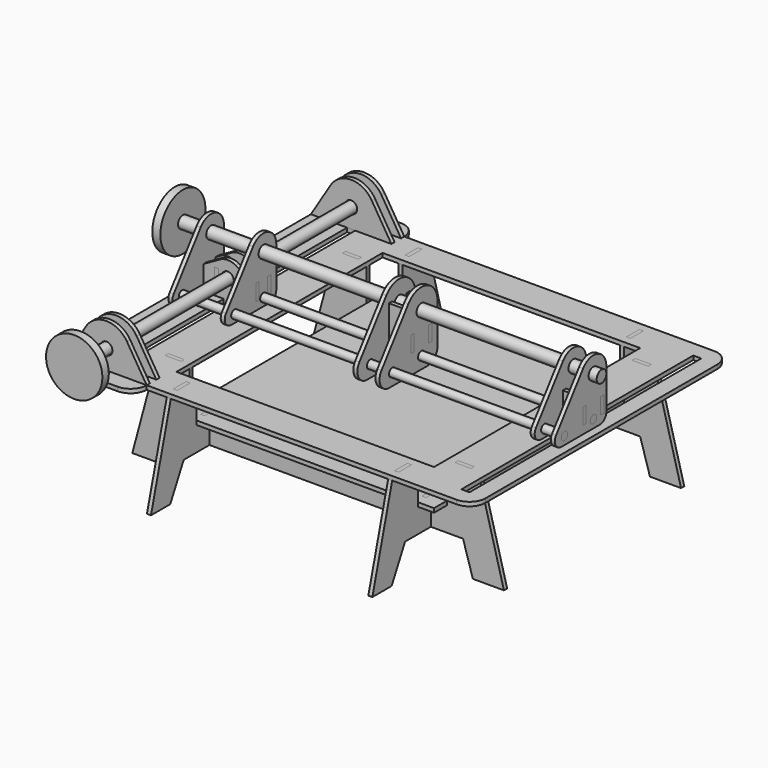
from build123d import *

# Parameters (mm, degrees)
F0_W           = 203.2
F0_H           = 203.2
F1_DEPTH       = 3.175
F3_W           = 203.2
F3_H           = 203.2
F4_DEPTH       = 3.175
F6_DEPTH       = 3.175
F10_DEPTH      = 3.175
F14_DEPTH      = 3.175
F7_W           = 6.35
F7_H           = 228.6
F16_DEPTH      = 8.128
F18_R          = 4.7625
F19_DEPTH      = 3.175
F25_R          = 3.175
F25_R_2        = 4.7625
F26_DEPTH      = 3.175
F30_R          = 4.7625
F31_DEPTH      = 3.175
F34_R          = 3.175
F34_R_2        = 4.7625
F35_DEPTH      = 3.175
F38_R          = 3.175
F39_DEPTH      = 146.05
F39_DEPTH_BACK = 158.75
F41_R          = 3.302
F41_R_2        = 4.7625
F42_DEPTH      = 3.175
F44_R          = 4.7625
F45_DEPTH      = 152.4
F45_DEPTH_BACK = 177.8
F46_R          = 4.4516956425
F47_DEPTH      = 152.4
F47_DEPTH_BACK = 133.35
F49_DEPTH      = 3.175
F51_R          = 22.225
F51_R_2        = 4.4516956425
F52_DEPTH      = 6.35
F53_R          = 22.225
F53_R_2        = 4.7625
F54_DEPTH      = 6.35
F55_W          = 3.175
F55_H          = 12.7
F56_DEPTH      = 3.175
F61_DEPTH      = 3.175
F63_W          = 3.175
F63_H          = 12.7
F63_W_2        = 12.7
F63_H_2        = 3.175
F64_DEPTH      = 25.4
F65_W          = 12.7
F65_H          = 3.175
F66_DEPTH      = 25.4
F67_W          = 3.175
F67_H          = 6.35
F68_DEPTH      = 25.4
F69_W          = 3.175
F69_H          = 12.7
F70_DEPTH      = 51.054
F71_W          = 3.175
F71_H          = 12.7
F72_DEPTH      = 25.4
F73_W          = 3.175
F73_H          = 12.7
F74_DEPTH      = 25.4
F76_DEPTH      = 25.4


with BuildPart() as f1:
    # F0 (on Top) → F1 (new body)
    with BuildSketch(Plane.XY):
        Rectangle(F0_W, F0_H)
    extrude(amount=-F1_DEPTH)

    # F75 (on face) → F76 (cut)
    with BuildSketch(Plane.XY):
        Polygon((-85.725, 88.9), (-85.725, 93.6625), (-88.9, 93.6625), (-88.9, 88.9), (-93.6625, 88.9), (-93.6625, 85.725), (-88.9, 85.725), (-88.9, 80.9625), (-85.725, 80.9625), (-85.725, 85.725), (-80.9625, 85.725), (-80.9625, 88.9), align=None)
        Polygon((88.9, 85.725), (93.6625, 85.725), (93.6625, 88.9), (88.9, 88.9), (88.9, 93.6625), (85.725, 93.6625), (85.725, 88.9), (80.9625, 88.9), (80.9625, 85.725), (85.725, 85.725), (85.725, 80.9625), (88.9, 80.9625), align=None)
        Polygon((-88.9, -88.9), (-88.9, -93.6625), (-85.725, -93.6625), (-85.725, -88.9), (-80.9625, -88.9), (-80.9625, -85.725), (-85.725, -85.725), (-85.725, -80.9625), (-88.9, -80.9625), (-88.9, -85.725), (-93.6625, -85.725), (-93.6625, -88.9), align=None)
        Polygon((85.725, -93.6625), (88.9, -93.6625), (88.9, -88.9), (93.6625, -88.9), (93.6625, -85.725), (88.9, -85.725), (88.9, -80.9625), (85.725, -80.9625), (85.725, -85.725), (80.9625, -85.725), (80.9625, -88.9), (85.725, -88.9), align=None)
    extrude(amount=-F76_DEPTH, mode=Mode.SUBTRACT)


with BuildPart() as f4:
    # F3 (on offset) → F4 (new body)
    with BuildSketch(Plane.XY.offset(25.4)):
        with BuildLine():
            Line((114.3, 127), (-114.3, 127))
            Line((-114.3, 127), (-139.7, 127))
            ThreePointArc((-139.7, 127), (-148.6802561211, 123.2802561211), (-152.4, 114.3))
            Line((-152.4, 114.3), (-152.4, 101.6))
            Line((-152.4, 101.6), (-152.4, -101.6))
            Line((-152.4, -101.6), (-152.4, -114.3))
            ThreePointArc((-152.4, -114.3), (-148.6802561211, -123.2802561211), (-139.7, -127))
            Line((-139.7, -127), (-114.3, -127))
            Line((-114.3, -127), (114.3, -127))
            Line((114.3, -127), (139.7, -127))
            ThreePointArc((139.7, -127), (148.6802561211, -123.2802561211), (152.4, -114.3))
            Line((152.4, -114.3), (152.4, -101.6))
            Line((152.4, -101.6), (152.4, 101.6))
            Line((152.4, 101.6), (152.4, 114.3))
            ThreePointArc((152.4, 114.3), (148.6802561211, 123.2802561211), (139.7, 127))
            Line((139.7, 127), (114.3, 127))
        make_face()
        Rectangle(F3_W, F3_H, mode=Mode.SUBTRACT)
    extrude(amount=F4_DEPTH)

    # F5 (on face) → F6 (join)
    with BuildSketch(Plane.XY.offset(28.575)):
        with BuildLine():
            ThreePointArc((-168.275, -127), (-164.5552561211, -135.9802561211), (-155.575, -139.7))
            Line((-155.575, -139.7), (-117.475, -139.7))
            ThreePointArc((-117.475, -139.7), (-108.4947438789, -135.9802561211), (-104.775, -127))
            Line((-104.775, -127), (-104.775, 127))
            ThreePointArc((-104.775, 127), (-108.4947438789, 135.9802561211), (-117.475, 139.7))
            Line((-117.475, 139.7), (-155.575, 139.7))
            ThreePointArc((-155.575, 139.7), (-164.5552561211, 135.9802561211), (-168.275, 127))
            Line((-168.275, 127), (-168.275, -127))
        make_face()
    extrude(amount=-F6_DEPTH)

    # F7 (on face) → F16 (cut)
    with BuildSketch(Plane.XY.offset(28.575)):
        with Locations((-136.525, 0)):
            Rectangle(F7_W, F7_H)
        with Locations((136.525, 0)):
            Rectangle(F7_W, F7_H)
    extrude(amount=-F16_DEPTH, mode=Mode.SUBTRACT)

    # F63 (on face) → F64 (cut)
    with BuildSketch(Plane.XY.offset(28.575)):
        with Locations((-87.3125, 114.3)):
            Rectangle(F63_W, F63_H)
        with Locations((-114.3, 87.3125)):
            Rectangle(F63_W_2, F63_H_2)
        with Locations((87.3125, 114.3)):
            Rectangle(F63_W, F63_H)
        with Locations((114.3, 87.3125)):
            Rectangle(F63_W_2, F63_H_2)
        with Locations((114.3, -87.3125)):
            Rectangle(F63_W_2, F63_H_2)
        with Locations((87.3125, -114.3)):
            Rectangle(F63_W, F63_H)
        with Locations((-87.3125, -114.3)):
            Rectangle(F63_W, F63_H)
        with Locations((-114.3, -87.3125)):
            Rectangle(F63_W_2, F63_H_2)
    extrude(amount=-F64_DEPTH, mode=Mode.SUBTRACT)

    # F65 (on face) → F66 (cut)
    with BuildSketch(Plane(origin=(0, 0, 25.4), x_dir=(1, 0, 0), z_dir=(0, 0, -1))):
        with Locations((-155.575, 125.4125)):
            Rectangle(F65_W, F65_H)
        with Locations((-155.575, 115.8875)):
            Rectangle(F65_W, F65_H)
        with Locations((-117.475, 125.4125)):
            Rectangle(F65_W, F65_H)
        with Locations((-117.475, 115.8875)):
            Rectangle(F65_W, F65_H)
        with Locations((-117.475, -115.8875)):
            Rectangle(F65_W, F65_H)
        with Locations((-117.475, -125.4125)):
            Rectangle(F65_W, F65_H)
        with Locations((-155.575, -125.4125)):
            Rectangle(F65_W, F65_H)
        with Locations((-155.575, -115.8875)):
            Rectangle(F65_W, F65_H)
    extrude(amount=-F66_DEPTH, mode=Mode.SUBTRACT)


with BuildPart() as f10:
    # F9 (on offset) → F10 (new body)
    with BuildSketch(Plane.YZ.offset(-88.9)):
        Polygon((80.9625, -3.175), (0, -3.175), (-80.9625, -3.175), (-80.9625, 0), (-93.6625, 0), (-93.6625, -3.175), (-101.6, -3.175), (-101.6, 0), (-101.6, 25.4), (-107.95, 25.4), (-107.95, 28.575), (-120.65, 28.575), (-120.65, 25.4), (-127, 25.4), (-146.5669897773, -47.625), (-127.5169897773, -47.625), (-114.3, -22.225), (-88.9, -22.225), (-88.9, -10.795), (-85.725, -10.795), (-85.725, -22.225), (0, -22.225), (85.725, -22.225), (85.725, -10.795), (88.9, -10.795), (88.9, -22.225), (114.3, -22.225), (127.5169897773, -47.625), (146.5669897773, -47.625), (127, 25.4), (120.65, 25.4), (120.65, 28.575), (107.95, 28.575), (107.95, 25.4), (101.6, 25.4), (101.6, 0), (101.6, -3.175), (93.6625, -3.175), (93.6625, 0), (80.9625, 0), align=None)
    extrude(amount=F10_DEPTH)


with BuildPart() as f11_1:
    # F11: instance of F10
    add(f10.part.mirror(Plane.YZ))


with BuildPart() as f14:
    # F13 (on offset) → F14 (new body)
    with BuildSketch(Plane.XZ.offset(88.9)):
        Polygon((-93.6625, -3.175), (-101.6, -3.175), (-101.6, 0), (-101.6, 25.4), (-107.95, 25.4), (-107.95, 28.575), (-120.65, 28.575), (-120.65, 25.4), (-127, 25.4), (-146.5669897773, -47.625), (-122.0367805193, -47.625), (-114.3, -22.225), (0, -22.225), (114.3, -22.225), (122.0367805193, -47.625), (146.5669897773, -47.625), (127, 25.4), (120.65, 25.4), (120.65, 28.575), (107.95, 28.575), (107.95, 25.4), (101.6, 25.4), (101.6, 0), (101.6, -3.175), (93.6625, -3.175), (93.6625, 0), (88.9, 0), (88.9, -11.43), (85.725, -11.43), (85.725, 0), (80.9625, 0), (80.9625, -3.175), (0, -3.175), (-80.9625, -3.175), (-80.9625, 0), (-85.725, 0), (-85.725, -11.43), (-88.9, -11.43), (-88.9, 0), (-93.6625, 0), align=None)
    extrude(amount=-F14_DEPTH)


with BuildPart() as f15_1:
    # F15: instance of F14
    add(f14.part.mirror(Plane.XZ))


with BuildPart() as f19:
    # F18 (on offset) → F19 (new body)
    with BuildSketch(Plane.XZ.offset(114.3)):
        with BuildLine():
            Line((-104.775, 28.575), (-120.3018889302, 53.800648062))
            ThreePointArc((-120.3018889302, 53.800648062), (-136.525, 62.865), (-152.7481110698, 53.800648062))
            Line((-152.7481110698, 53.800648062), (-168.275, 28.575))
            Line((-168.275, 28.575), (-161.925, 28.575))
            Line((-161.925, 28.575), (-161.925, 25.4))
            Line((-161.925, 25.4), (-149.225, 25.4))
            Line((-149.225, 25.4), (-149.225, 28.575))
            Line((-149.225, 28.575), (-123.825, 28.575))
            Line((-123.825, 28.575), (-123.825, 25.4))
            Line((-123.825, 25.4), (-111.125, 25.4))
            Line((-111.125, 25.4), (-111.125, 28.575))
            Line((-111.125, 28.575), (-104.775, 28.575))
        make_face()
        with Locations((-136.525, 43.815)):
            Circle(F18_R, mode=Mode.SUBTRACT)
    extrude(amount=F19_DEPTH)


with BuildPart() as f21_1:
    # F21: instance of F19
    add(f19.part.mirror(Plane.XZ.offset(120.65)))


with BuildPart() as f22_1:
    # F22: instance of F21_1
    add(f21_1.part.mirror(Plane.XZ))


with BuildPart() as f22_2:
    # F22: instance of F19
    add(f19.part.mirror(Plane.XZ))


with BuildPart() as f26:
    # F25 (on offset) → F26 (new body)
    with BuildSketch(Plane.YZ.offset(-114.3)):
        with BuildLine():
            Line((12.7, 34.925), (12.7, 66.675))
            ThreePointArc((12.7, 66.675), (4.0160926284, 78.7232778852), (-10.16, 74.295))
            Line((-10.16, 74.295), (-36.83, 38.735))
            ThreePointArc((-36.83, 38.735), (-37.4296126628, 32.0851936686), (-31.75, 28.575))
            Line((-31.75, 28.575), (6.35, 28.575))
            ThreePointArc((6.35, 28.575), (10.8401280605, 30.4348719395), (12.7, 34.925))
        make_face()
        with Locations((-28.575, 34.925)):
            Circle(F25_R, mode=Mode.SUBTRACT)
        with Locations((0, 34.925)):
            Circle(F25_R, mode=Mode.SUBTRACT)
        with Locations((0, 66.675)):
            Circle(F25_R_2, mode=Mode.SUBTRACT)
    extrude(amount=-F26_DEPTH)


with BuildPart() as f27_1:
    # F27: instance of F26
    add(f26.part.mirror(Plane.YZ.offset(-136.525)))


with BuildPart() as f31:
    # F30 (on offset) → F31 (new body)
    with BuildSketch(Plane.XZ.offset(4.1656)):
        with BuildLine():
            Line((-155.575, 34.925), (-155.575, 28.575))
            Line((-155.575, 28.575), (-139.7, 28.575))
            Line((-139.7, 28.575), (-139.7, 25.4))
            Line((-139.7, 25.4), (-133.35, 25.4))
            Line((-133.35, 25.4), (-133.35, 28.575))
            Line((-133.35, 28.575), (-117.475, 28.575))
            Line((-117.475, 28.575), (-117.475, 34.925))
            Line((-117.475, 34.925), (-114.3, 34.925))
            Line((-114.3, 34.925), (-114.3, 47.625))
            Line((-114.3, 47.625), (-117.475, 47.625))
            Line((-117.475, 47.625), (-130.2687580598, 54.8671236324))
            ThreePointArc((-130.2687580598, 54.8671236324), (-136.525, 56.515), (-142.7812419402, 54.8671236324))
            Line((-142.7812419402, 54.8671236324), (-155.575, 47.625))
            Line((-155.575, 47.625), (-158.75, 47.625))
            Line((-158.75, 47.625), (-158.75, 34.925))
            Line((-158.75, 34.925), (-155.575, 34.925))
        make_face()
        with Locations((-136.525, 43.815)):
            Circle(F30_R, mode=Mode.SUBTRACT)
    extrude(amount=F31_DEPTH)


with BuildPart() as f32_1:
    # F32: instance of F31
    add(f31.part.mirror(Plane.XZ))


with BuildPart() as f35:
    # F34 (on offset) → F35 (new body)
    with BuildSketch(Plane.YZ.offset(127)):
        with BuildLine():
            Line((12.7, 34.925), (12.7, 66.675))
            ThreePointArc((12.7, 66.675), (4.0160926284, 78.7232778852), (-10.16, 74.295))
            Line((-10.16, 74.295), (-36.83, 38.735))
            ThreePointArc((-36.83, 38.735), (-37.4296126628, 32.0851936686), (-31.75, 28.575))
            Line((-31.75, 28.575), (6.35, 28.575))
            ThreePointArc((6.35, 28.575), (10.8401280605, 30.4348719395), (12.7, 34.925))
        make_face()
        with Locations((-28.575, 34.925)):
            Circle(F34_R, mode=Mode.SUBTRACT)
        with Locations((0, 34.925)):
            Circle(F34_R, mode=Mode.SUBTRACT)
        with Locations((0, 66.675)):
            Circle(F34_R_2, mode=Mode.SUBTRACT)
    extrude(amount=F35_DEPTH)


with BuildPart() as f37_1:
    # F37: instance of F35
    add(f35.part.mirror(Plane.YZ.offset(136.525)))


with BuildPart() as f39:
    # F38 (on Right) → F39 (new body, two sides)
    with BuildSketch(Plane.YZ) as f39_sk:
        with Locations((-28.575, 34.925)):
            Circle(F38_R)
    extrude(amount=F39_DEPTH)
    extrude(f39_sk.sketch, amount=-F39_DEPTH_BACK)


with BuildPart() as f39b:
    # F38 (on Right) → F39, piece 2 (new body, two sides)
    with BuildSketch(Plane.YZ) as f39_2_sk:
        with Locations((0, 34.925)):
            Circle(F38_R)
    extrude(amount=F39_DEPTH)
    extrude(f39_2_sk.sketch, amount=-F39_DEPTH_BACK)


with BuildPart() as f42:
    # F41 (on offset) → F42 (new body)
    with BuildSketch(Plane.YZ.offset(7.14375)):
        with BuildLine():
            Line((15.875, 34.925), (15.875, 66.675))
            ThreePointArc((15.875, 66.675), (5.0201157855, 81.7353473566), (-12.7, 76.2))
            Line((-12.7, 76.2), (-39.37, 40.64))
            ThreePointArc((-39.37, 40.64), (-40.2694189943, 30.6652905029), (-31.75, 25.4))
            Line((-31.75, 25.4), (6.35, 25.4))
            ThreePointArc((6.35, 25.4), (13.0851920908, 28.1898079092), (15.875, 34.925))
        make_face()
        with Locations((-28.575, 34.925)):
            Circle(F41_R, mode=Mode.SUBTRACT)
        with Locations((0, 34.925)):
            Circle(F41_R, mode=Mode.SUBTRACT)
        with Locations((0, 66.675)):
            Circle(F41_R_2, mode=Mode.SUBTRACT)
    extrude(amount=F42_DEPTH)


with BuildPart() as f43_1:
    # F43: instance of F42
    add(f42.part.mirror(Plane.YZ))


with BuildPart() as f45:
    # F44 (on Right) → F45 (new body, two sides)
    with BuildSketch(Plane.YZ) as f45_sk:
        with Locations((0, 66.675)):
            Circle(F44_R)
    extrude(amount=F45_DEPTH)
    extrude(f45_sk.sketch, amount=-F45_DEPTH_BACK)

    # F53 (on face) → F54 (join)
    with BuildSketch(Plane(origin=(-177.8, 0, 0), x_dir=(0, -1, 0), z_dir=(-1, 0, 0))):
        with Locations((0, 66.675)):
            Circle(F53_R)
        with Locations((0, 66.675)):
            Circle(F53_R_2, mode=Mode.SUBTRACT)
        with Locations((0, 66.675)):
            Circle(F53_R_2)
    extrude(amount=F54_DEPTH)


with BuildPart() as f47:
    # F46 (on Front) → F47 (new body, two sides)
    with BuildSketch(Plane.XZ) as f47_sk:
        with Locations((-136.525, 43.815)):
            Circle(F46_R)
    extrude(amount=F47_DEPTH)
    extrude(f47_sk.sketch, amount=-F47_DEPTH_BACK)

    # F51 (on face) → F52 (join)
    with BuildSketch(Plane.XZ.offset(152.4)):
        with Locations((-136.525, 43.815)):
            Circle(F51_R)
        with Locations((-136.525, 43.815)):
            Circle(F51_R_2, mode=Mode.SUBTRACT)
        with Locations((-136.525, 43.815)):
            Circle(F51_R_2)
    extrude(amount=F52_DEPTH)


with BuildPart() as f49:
    # F48 (on offset) → F49 (new body)
    with BuildSketch(Plane.XZ.offset(7.14375)):
        Polygon((142.875, 53.975), (130.175, 53.975), (130.175, 47.625), (127, 47.625), (127, 34.925), (130.175, 34.925), (130.175, 28.575), (133.477, 28.575), (133.477, 25.4), (139.573, 25.4), (139.573, 28.575), (142.875, 28.575), (142.875, 34.925), (146.05, 34.925), (146.05, 47.625), (142.875, 47.625), align=None)
    extrude(amount=F49_DEPTH)


with BuildPart() as f50_1:
    # F50: instance of F49
    add(f49.part.mirror(Plane.XZ))


with BuildPart() as f56:
    # F55 (on offset) → F56 (new body)
    with BuildSketch(Plane.XZ.offset(7.14375)):
        Polygon((7.14375, 69.85), (-7.14375, 69.85), (-7.14375, 53.34), (-7.14375, 40.64), (-7.14375, 31.75), (7.14375, 31.75), (7.14375, 40.64), (7.14375, 53.34), align=None)
        with Locations((-8.73125, 46.99)):
            Rectangle(F55_W, F55_H)
        with Locations((8.73125, 46.99)):
            Rectangle(F55_W, F55_H)
    extrude(amount=F56_DEPTH)


with BuildPart() as f57_1:
    # F57: instance of F56
    add(f56.part.mirror(Plane.XZ))


with BuildPart() as f61:
    # F60 (on offset) → F61 (new body)
    with BuildSketch(Plane.YZ.offset(-129.38125)):
        Polygon((4.1656, 48.26), (4.1656, 51.435), (-4.1656, 51.435), (-4.1656, 48.26), (-7.3406, 48.26), (-7.3406, 41.91), (-4.1656, 41.91), (-4.1656, 38.735), (4.1656, 38.735), (4.1656, 41.91), (7.3406, 41.91), (7.3406, 48.26), align=None)
    extrude(amount=F61_DEPTH)


with BuildPart() as f62_1:
    # F62: instance of F61
    add(f61.part.mirror(Plane.YZ.offset(-136.525)))


with BuildPart() as f68_tool:
    # F67 (on face) → F68 (new body)
    with BuildSketch(Plane.XZ.offset(7.3406)):
        with Locations((-145.25625, 45.085)):
            Rectangle(F67_W, F67_H)
        with Locations((-127.79375, 45.085)):
            Rectangle(F67_W, F67_H)
    extrude(amount=-F68_DEPTH)


with BuildPart() as f31_1:
    add(f31.part)

    # F68: cut by f68_tool
    add(f68_tool.part, mode=Mode.SUBTRACT)


with BuildPart() as f32_1_1:
    add(f32_1.part)

    # F68: cut by f68_tool
    add(f68_tool.part, mode=Mode.SUBTRACT)


with BuildPart() as f70_tool:
    # F69 (on face) → F70 (new body)
    with BuildSketch(Plane(origin=(-158.75, 0, 0), x_dir=(0, -1, 0), z_dir=(-1, 0, 0))):
        with Locations((5.7531, 41.275)):
            Rectangle(F69_W, F69_H)
        with Locations((-5.7531, 41.275)):
            Rectangle(F69_W, F69_H)
    extrude(amount=-F70_DEPTH)


with BuildPart() as f26_1:
    add(f26.part)

    # F70: cut by f70_tool
    add(f70_tool.part, mode=Mode.SUBTRACT)


with BuildPart() as f27_1_1:
    add(f27_1.part)

    # F70: cut by f70_tool
    add(f70_tool.part, mode=Mode.SUBTRACT)


with BuildPart() as f72_tool:
    # F71 (on face) → F72 (new body)
    with BuildSketch(Plane(origin=(-10.31875, 0, 0), x_dir=(0, -1, 0), z_dir=(-1, 0, 0))):
        with Locations((8.73125, 46.99)):
            Rectangle(F71_W, F71_H)
        with Locations((-8.73125, 46.99)):
            Rectangle(F71_W, F71_H)
    extrude(amount=-F72_DEPTH)


with BuildPart() as f42_1:
    add(f42.part)

    # F72: cut by f72_tool
    add(f72_tool.part, mode=Mode.SUBTRACT)


with BuildPart() as f43_1_1:
    add(f43_1.part)

    # F72: cut by f72_tool
    add(f72_tool.part, mode=Mode.SUBTRACT)


with BuildPart() as f74_tool:
    # F73 (on face) → F74 (new body)
    with BuildSketch(Plane.YZ.offset(146.05)):
        with Locations((-8.73125, 41.275)):
            Rectangle(F73_W, F73_H)
        with Locations((8.73125, 41.275)):
            Rectangle(F73_W, F73_H)
    extrude(amount=-F74_DEPTH)


with BuildPart() as f35_1:
    add(f35.part)

    # F74: cut by f74_tool
    add(f74_tool.part, mode=Mode.SUBTRACT)


with BuildPart() as f37_1_1:
    add(f37_1.part)

    # F74: cut by f74_tool
    add(f74_tool.part, mode=Mode.SUBTRACT)


solid = Compound([f1.part, f4.part, f10.part, f11_1.part, f14.part, f15_1.part, f19.part, f21_1.part, f22_1.part, f22_2.part, f39.part, f39b.part, f45.part, f47.part, f49.part, f50_1.part, f56.part, f57_1.part, f61.part, f62_1.part, f31_1.part, f32_1_1.part, f26_1.part, f27_1_1.part, f42_1.part, f43_1_1.part, f35_1.part, f37_1_1.part])
